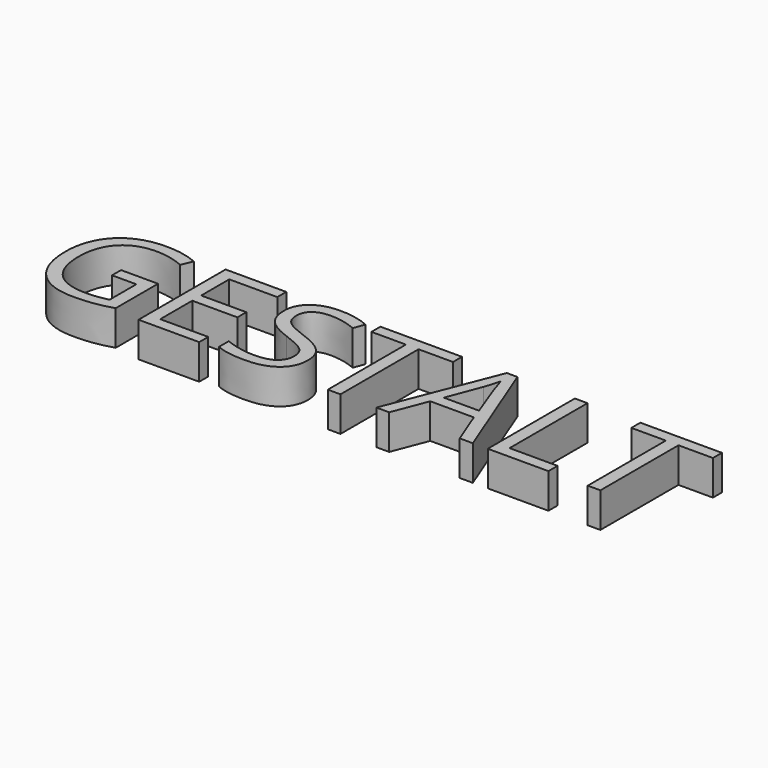
from build123d import *

# Parameters (mm, degrees)
F0_TEXT_SIZE = 45.4282646792
F1_DEPTH     = 10.4


# Not quite as in the source:
# - Text() gives the source's letters only with a copy of the font that has no kerning and outlines rounded to 1/6400 em; it was checked with that copy


with BuildPart() as f1:
    # F0 (on Top) → F1 (new body)
    with BuildSketch(Plane.XY):
        with Locations((-46.3195629418, -50.1478686929)):
            Text('GESTALT', F0_TEXT_SIZE, font='Open Sans', text_align=(TextAlign.LEFT, TextAlign.BOTTOM))
    extrude(amount=F1_DEPTH)


solid = f1.part
